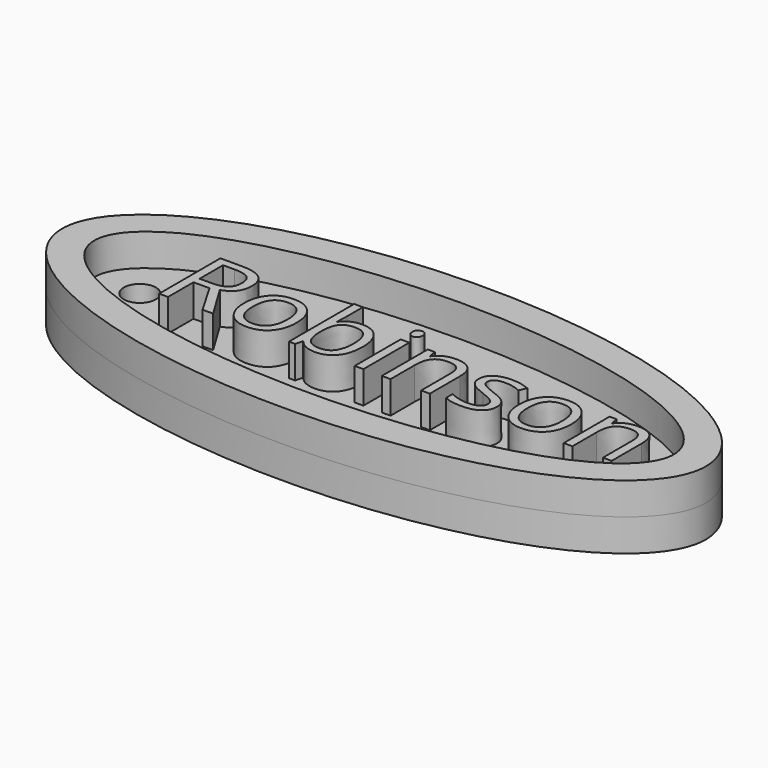
from build123d import *

# Parameters (mm, degrees)
F1_DEPTH     = 3.175
F3_DEPTH     = 3.175
F4_TEXT_SIZE = 10.5833333333
F5_DEPTH     = 3.175
F6_R         = 1.5875
F7_DEPTH     = 3.1760001


# Not quite as in the source:
# - a feature names something its author has since deleted; it is built from what else it names
# - Text() gives the source's letters only with a copy of the font that has no kerning and outlines rounded to 1/6400 em; it was checked with that copy


with BuildPart() as f1:
    # F0 (on Top) → F1 (new body, symmetric)
    with BuildSketch(Plane.XY):
        with BuildLine():
            add(Edge.make_bspline(
                [(31.75, 0), (31.75, 21.9970452561), (-15.875, 10.9985226281), (-63.5, 0), (-15.875, -10.9985226281), (31.75, -21.9970452561), (31.75, 0)],
                knots=[0, 0, 0, 2.0943951024, 2.0943951024, 4.1887902048, 4.1887902048, 6.2831853072, 6.2831853072, 6.2831853072], degree=2, weights=[1, 0.5, 1, 0.5, 1, 0.5, 1]))
        make_face()
    extrude(amount=F1_DEPTH, both=True)

    # F2 (on face) → F3 (cut)
    with BuildSketch(Plane.XY.offset(3.175)):
        with BuildLine():
            add(Edge.make_bspline(
                [(28.575, 0), (28.575, 16.4977839421), (-14.2875, 8.248891971), (-57.15, 0), (-14.2875, -8.248891971), (28.575, -16.4977839421), (28.575, 0)],
                knots=[0, 0, 0, 2.0943951024, 2.0943951024, 4.1887902048, 4.1887902048, 6.2831853072, 6.2831853072, 6.2831853072], degree=2, weights=[1, 0.5, 1, 0.5, 1, 0.5, 1]))
        make_face()
    extrude(amount=-F3_DEPTH, mode=Mode.SUBTRACT)

    # F4 (on face) → F5 (join)
    with BuildSketch(Plane.XY):
        with Locations((-20.1755017783, -3.81)):
            Text('Robinson', F4_TEXT_SIZE, font='Open Sans', text_align=(TextAlign.LEFT, TextAlign.BOTTOM))
    extrude(amount=F5_DEPTH)

    # F6 (on face) → F7 (cut, through all)
    with BuildSketch(Plane.XY):
        with Locations((-24.13, 0.0548721582)):
            Circle(F6_R)
    extrude(amount=-F7_DEPTH, mode=Mode.SUBTRACT)


solid = f1.part
